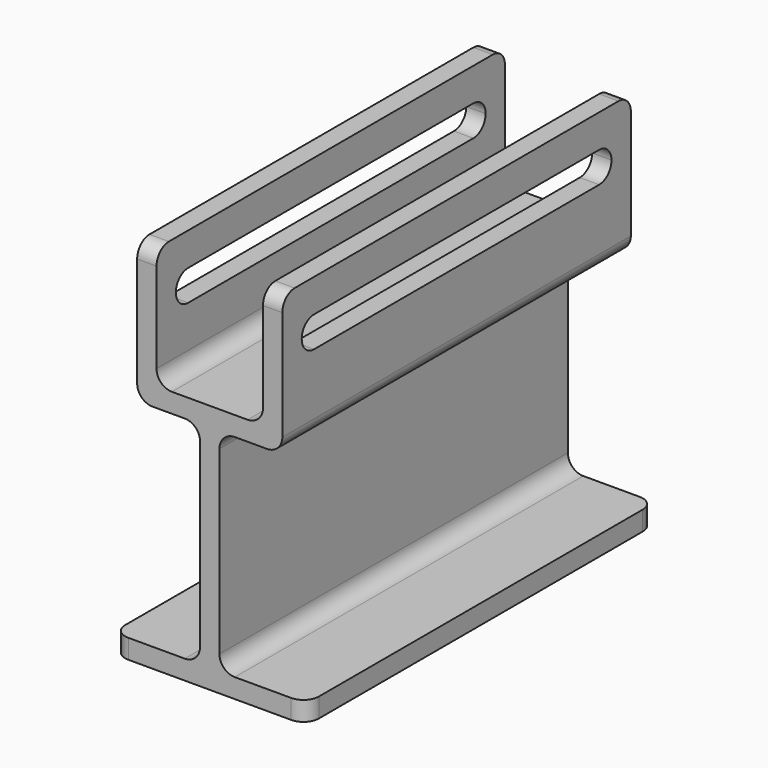
from build123d import *

# Parameters (mm, degrees)
F0_W     = 4
F0_H     = 4
F0_H_2   = 6
F1_DEPTH = 90
F2_W     = 80
F2_H     = 6.35
F3_DEPTH = 25
F4_R     = 3.17499


# Not quite as in the source:
# - a fillet or chamfer is up to 0.001 mm smaller than in the source, because OpenCascade refuses the exact size


with BuildPart() as f1:
    # F0 (on Front) → F1 (new body)
    with BuildSketch(Plane.XZ):
        with Locations((-13, 27)):
            Rectangle(F0_W, F0_H)
        with Locations((-13, 22)):
            Rectangle(F0_W, F0_H_2)
        Polygon((-11, 19), (-15, 19), (-15, 0), (-2, 0), (-2, -43.675), (-20, -43.675), (-20, -47.675), (0, -47.675), (0, 0), (0, 4), (-11, 4), align=None)
    extrude(amount=F1_DEPTH)

    # F2 (on face) → F3 (cut)
    with BuildSketch(Plane(origin=(-15, 0, 0), x_dir=(0, -1, 0), z_dir=(-1, 0, 0))):
        with Locations((45, 19)):
            Rectangle(F2_W, F2_H)
    extrude(amount=-F3_DEPTH, mode=Mode.SUBTRACT)

    # F4 (radius 3.175 in the source; OpenCascade refuses exactly that, so slightly less here)
    f4_edges = [f1.edges().sort_by_distance(p)[0] for p in [
        (-13, 0, 29),
        (-13, -90, 29),
        (-11, -45, 4),
        (-15, -45, 0),
        (-20, 0, -45.675),
        (-20, -90, -45.675),
        (-13, -85, 22.175),
        (-13, -85, 15.825),
        (-13, -5, 15.825),
        (-13, -5, 22.175),
        (-2, -45, -43.675),
        (-2, -45, 0),
    ]]
    fillet(f4_edges, radius=F4_R)

    # F5: F1 across plane


with BuildPart() as f1_1:
    add(f1.part)
    add(f1.part.mirror(Plane.YZ))


solid = f1_1.part
